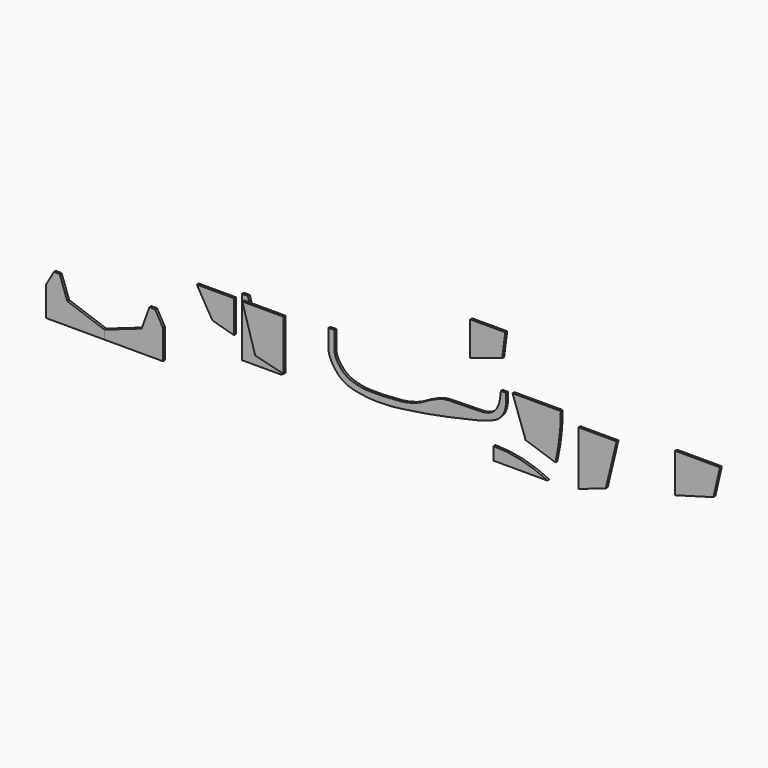
from build123d import *

# Parameters (mm, degrees)
F3_DEPTH  = 6
F6_DEPTH  = 6
F9_DEPTH  = 6
F11_ANGLE = -90


# Not quite as in the source:
# - the dataset's text gives a spline's control points without its knots; the knots are read off the source's solid


with BuildPart() as f3:
    # F2 (on offset) → F3 (new body, symmetric)
    with BuildSketch(Plane.XZ.offset(150)):
        Polygon((-3625.609999, -171.762304), (-3690.988803, 14.456954), (-3734.999999, 14.456954), (-3734.999999, -278.043046), (-3587.000738, -278.043046), (-3518.834227, -239.119074), (-3518.737431, -210.119236), align=None)
    extrude(amount=F3_DEPTH, both=True)


with BuildPart() as f3b:
    # F2 (on offset) → F3, piece 2 (new body, symmetric)
    with BuildSketch(Plane.XZ.offset(150)):
        Polygon((-3499.359797, 15.171997), (-3685.363609, 15.171997), (-3607.548165, -117.352554), (-3499.359797, -147.688624), align=None)
    extrude(amount=F3_DEPTH, both=True)


with BuildPart() as f3c:
    # F2 (on offset) → F3, piece 3 (new body, symmetric)
    with BuildSketch(Plane.XZ.offset(150)):
        Polygon((-3392.94012, -202.496046), (-3250.269731, -237.505348), (-3250.269731, 14.456954), (-3457.53672, 14.456954), align=None)
    extrude(amount=F3_DEPTH, both=True)


with BuildPart() as f3d:
    # F2 (on offset) → F3, piece 4 (new body, symmetric)
    with BuildSketch(Plane.XZ.offset(150)):
        with BuildLine():
            Line((-2039.001766, -135.293519), (-1889.685851, -184.798644))
            ThreePointArc((-1889.6858509731, -184.7986440063), (-1869.4967950194, -68.0992181167), (-1862.9039386122, 50.150045))
            Line((-1862.9039386122, 50.150045), (-2104.665183, 50.150045))
            Line((-2104.665183, 50.150045), (-2039.001766, -135.293519))
        make_face()
    extrude(amount=F3_DEPTH, both=True)


with BuildPart() as f3e:
    # F2 (on offset) → F3, piece 5 (new body, symmetric)
    with BuildSketch(Plane.XZ.offset(150)):
        Polygon((-1775.168843, -264.738794), (-1637.578437, -217.067599), (-1583.677871, 7.199494), (-1775.168843, 7.199494), align=None)
    extrude(amount=F3_DEPTH, both=True)


with BuildPart() as f3f:
    # F2 (on offset) → F3, piece 6 (new body, symmetric)
    with BuildSketch(Plane.XZ.offset(150)):
        Polygon((-1065.832633, 60.966433), (-1290.957958, 61.2627047565), (-1290.957958, -134.746592), (-1098.645907, -80.847844), align=None)
    extrude(amount=F3_DEPTH, both=True)


with BuildPart() as f3g:
    # F2 (on offset) → F3, piece 7 (new body, symmetric)
    with BuildSketch(Plane.XZ.offset(150)):
        Polygon((-2316.415245, 137.458014), (-2156.264262, 187.981895), (-2140.910383, 306.936754), (-2316.415245, 306.936754), align=None)
    extrude(amount=F3_DEPTH, both=True)


with BuildPart() as f3h:
    # F2 (on offset) → F3, piece 8 (new body, symmetric)
    with BuildSketch(Plane.XZ.offset(150)):
        with BuildLine():
            Line((-2199.840368, -278.0430460122), (-1929.8403680061, -278.0430460122))
            ThreePointArc((-1929.8403680061, -278.0430460122), (-2061.0784852524, -230.1263870226), (-2199.840368, -213.860179))
            Line((-2199.840368, -213.860179), (-2199.840368, -278.0430460122))
        make_face()
    extrude(amount=F3_DEPTH, both=True)


with BuildPart() as f6:
    # F5 (on offset) → F6 (new body, symmetric)
    with BuildSketch(Plane.XZ.offset(100)):
        Polygon((-3401.608404, -206.874181), (-3469.538726, 14.456954), (-3499.044418335, 14.456954), (-3499.044418335, -277.9286801815), (-3301.020689, -278.043046), (-3301.72565, -231.357552), align=None)
    extrude(amount=F6_DEPTH, both=True)


with BuildPart() as f9:
    # F8 (on offset) → F9 (new body, symmetric)
    with BuildSketch(Plane.XZ.offset(50)):
        with BuildLine():
            Line((-3075.793183, -27.575335), (-3106.845271, -28.364036))
            add(Edge.make_bspline(
                [(-3106.845271, -28.364036), (-3106.840775, -36.20769), (-3106.828893, -56.932157), (-3105.836512, -88.160314), (-3107.713614, -120.623454), (-3102.153065, -149.910737), (-3089.809329, -175.720614), (-3073.12758, -199.871045), (-3055.10971, -222.072588), (-3032.293265, -238.618807), (-3007.37903, -252.168496), (-2977.490107, -261.521539), (-2943.159085, -267.164316), (-2905.313231, -272.48649), (-2866.732897, -274.749636), (-2827.374006, -272.886322), (-2787.986153, -272.231794), (-2748.44303, -266.719692), (-2708.767862, -261.206991), (-2658.879402, -254.180345), (-2600.285762, -244.605599), (-2529.648341, -230.58561), (-2462.645441, -217.07781), (-2398.621762, -202.286051), (-2346.260264, -189.924976), (-2305.080707, -177.280982), (-2275.977732, -165.332874), (-2254.962384, -153.276426), (-2241.280852, -138.294535), (-2229.938497, -121.980888), (-2221.468545, -100.848936), (-2216.655886, -76.679761), (-2216.562975, -50.550788), (-2216.420433, -34.191666), (-2216.34339, -25.34977)],
                knots=[0, 0, 0, 0, 23.529089, 62.168447, 93.743754, 120.743754, 150.576622, 178.80781, 208.824473, 235.731721, 262.750233, 293.637123, 329.105419, 367.052751, 408.283807, 444.780382, 485.227879, 526.337489, 564.390084, 605.438835, 677.466608, 742.466608, 821.472937, 882.505715, 939.584608, 982.874329, 1011.509971, 1033.982176, 1054.790828, 1071.761391, 1093.394699, 1122.549458, 1145.110487, 1171.647175, 1171.647175, 1171.647175, 1171.647175], degree=3))
            Line((-2216.34339, -25.34977), (-2243.053473, -25.436439))
            add(Edge.make_bspline(
                [(-2243.053473, -25.436439), (-2243.916857, -34.460192), (-2245.84715, -54.634861), (-2251.343152, -85.496062), (-2265.471169, -115.566346), (-2292.728638, -140.078464), (-2330.982203, -148.955251), (-2371.607509, -149.143447), (-2408.800033, -149.346579), (-2442.964948, -151.021595), (-2475.096892, -150.378407), (-2506.727498, -151.370557), (-2538.586552, -155.662034), (-2566.27765, -166.85753), (-2592.904658, -178.474234), (-2618.538052, -191.702367), (-2644.925712, -208.390999), (-2678.453392, -220.339913), (-2714.292579, -230.648605), (-2753.933288, -235.550875), (-2794.770536, -237.78102), (-2839.221606, -241.053851), (-2883.282404, -240.236258), (-2925.320342, -240.484472), (-2962.990807, -232.205691), (-2994.870552, -223.392259), (-3020.337283, -209.419157), (-3039.100911, -193.654759), (-3053.589507, -174.028448), (-3068.637463, -153.572569), (-3076.653841, -124.924129), (-3076.765311, -90.713948), (-3075.89377, -57.520386), (-3075.821733, -36.074835), (-3075.793183, -27.575335)],
                knots=[0, 0, 0, 0, 27.202941, 60.818414, 93.620853, 125.005562, 167.195608, 207.643105, 247.266331, 278.666968, 310.242275, 343.618913, 373.635575, 406.023845, 432.707173, 460.867428, 492.490205, 526.031225, 567.140834, 604.194849, 645.498602, 689.905808, 737.759753, 777.784745, 815.480899, 853.070791, 876.50154, 902.114037, 925.820576, 949.590305, 977.75056, 1013.105899, 1051.938875, 1077.433973, 1077.433973, 1077.433973, 1077.433973], degree=3))
        make_face()
    extrude(amount=F9_DEPTH, both=True)


with BuildPart() as f3_1:
    # F10: moved
    add(f3.part.moved(Location((0, -150, 0))))


with BuildPart() as f3_2:
    # F11: moved
    add(f3_1.part.rotate(Axis((-3734.999999, -300, -278.043046), (0, 1, 0)), F11_ANGLE))


with BuildPart() as f12_1:
    # F12: instance of F3
    add(f3_2.part.mirror(Plane(origin=(-4027.499999, -300, -256.037448), x_dir=(0, -1, 0), z_dir=(-1, 0, 0))))


solid = Compound([f3b.part, f3c.part, f3d.part, f3e.part, f3f.part, f3g.part, f3h.part, f6.part, f9.part, f3_2.part, f12_1.part])
